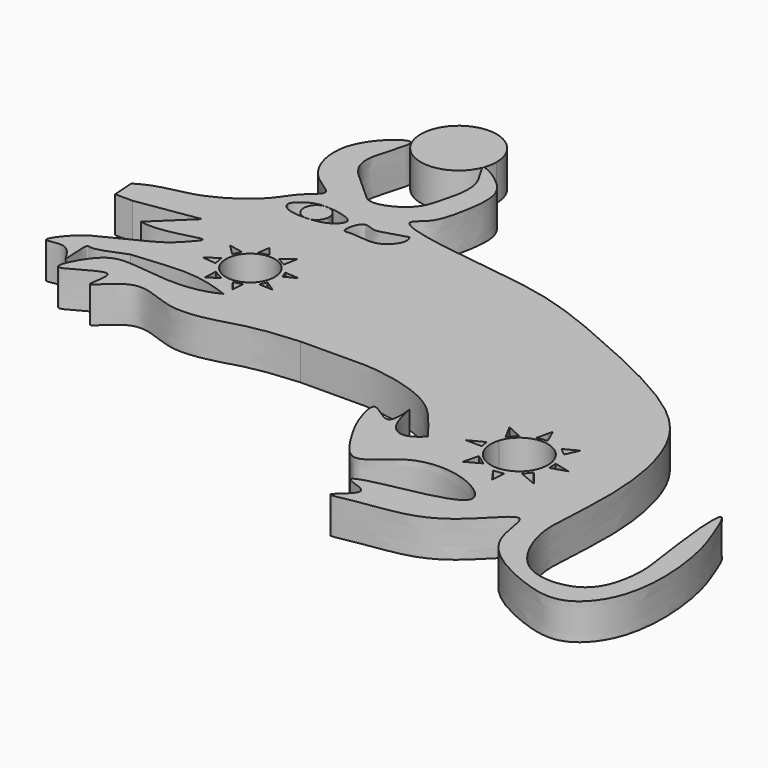
from build123d import *

# Parameters (mm, degrees)
F1_DEPTH = 6.35


with BuildPart() as f1:
    # F0 (on Top) → F1 (new body)
    with BuildSketch(Plane.XY):
        with BuildLine():
            Line((-51.3051622598, 40.6323485076), (-40.4214509814, 42.3343013825))
            Line((-40.4214509814, 42.3343013825), (-46.5386495977, 36.4676751196))
            add(Edge.make_bspline(
                [(-41.5301586996, 27.9514516536), (-43.7644399762, 26.9904386594), (-47.1679695554, 25.6974008069), (-48.0404193502, 26.9466699448), (-47.828587647, 22.82574291), (-47.5278895257, 20.4771889862), (-49.6106092059, 25.4928087476), (-54.8971564778, 22.8735531834), (-51.0068516627, 28.0945899918), (-48.0600885999, 29.6078924967), (-40.1052119231, 33.3394005284), (-38.1358371068, 35.4865499838), (-34.685151176, 39.2845987007), (-42.3593159189, 35.5881020627), (-46.5386495977, 36.4676751196)],
                knots=[0.9023541068, 0.9023541068, 0.9023541068, 0.9023541068, 0.907742959, 0.9125923743, 0.9207853725, 0.9255156021, 0.9337227858, 0.9415669865, 0.9501071173, 0.9590890143, 0.9716437394, 0.9798509262, 0.9862020834, 1, 1, 1, 1], degree=3))
            add(Edge.make_bspline(
                [(-29.9900722132, 33.1400264372), (-34.0198383076, 31.375468556), (-38.2517401569, 29.3615708058), (-41.5301586996, 27.9514516536)],
                knots=[0.8944469051, 0.8944469051, 0.8944469051, 0.8944469051, 0.9023541068, 0.9023541068, 0.9023541068, 0.9023541068], degree=3))
            ThreePointArc((-29.9900722132, 33.1400264372), (-27.7145464501, 39.0940051535), (-22.0091523445, 36.2521117437))
            add(Edge.make_bspline(
                [(-21.3412356287, 36.4475622498), (-21.5580775748, 36.3872225734), (-21.7808652609, 36.3219625695), (-22.0091523444, 36.2521117437)],
                knots=[0.8881591208, 0.8881591208, 0.8881591208, 0.8881591208, 0.8887349681, 0.8887349681, 0.8887349681, 0.8887349681], degree=3))
            Line((-21.3412356287, 36.4475622498), (-21.5400233865, 37.0286330581))
            Line((-21.5400233865, 37.0286330581), (-19.307261154, 36.8855050234))
            add(Edge.make_bspline(
                [(-24.2429566621, 26.7680510879), (-19.3063256589, 29.3490797871), (-14.3387897829, 36.8000169307), (-18.5226528543, 36.9870303006), (-19.307261154, 36.8855050234)],
                knots=[0.8683372636, 0.8683372636, 0.8683372636, 0.8683372636, 0.8834903862, 0.8861495586, 0.8861495586, 0.8861495586, 0.8861495586], degree=3))
            add(Edge.make_bspline(
                [(-7.1130855992, 22.3077908158), (-14.0992043325, 21.8413981828), (-17.6578918044, 20.5122390981), (-27.9317556959, 18.0093599196), (-35.5915896348, 23.5671974151), (-41.853535587, 14.694872303), (-38.2791283301, 24.7989362682), (-49.4655741655, 15.64594504), (-44.996041368, 24.6964345517), (-40.4360164412, 27.0000948649), (-29.9614893405, 23.7782191659), (-24.2429566621, 26.7680510879)],
                knots=[0.7600357456, 0.7600357456, 0.7600357456, 0.7600357456, 0.7751449316, 0.7881314628, 0.800745068, 0.8109455646, 0.8194731054, 0.8310040323, 0.8407808579, 0.8507840727, 0.8683372636, 0.8683372636, 0.8683372636, 0.8683372636], degree=3))
            add(Edge.make_bspline(
                [(36.6513938062, 22.1665031366), (25.3446848612, 23.1486310632), (3.3868181206, 23.0087634058), (-7.1130855992, 22.3077908158)],
                knots=[0.7373271423, 0.7373271423, 0.7373271423, 0.7373271423, 0.7600357456, 0.7600357456, 0.7600357456, 0.7600357456], degree=3))
            Line((36.6513938062, 22.1665031366), (36.8404947221, 22.9985490441))
            Line((36.8404947221, 22.9985490441), (37.2272023111, 22.1146447852))
            add(Edge.make_bspline(
                [(43.3149506831, 20.9869989592), (42.4581897705, 21.4586118414), (40.2700373504, 21.8304625428), (37.2272023111, 22.1146447852)],
                knots=[0.7306147118, 0.7306147118, 0.7306147118, 0.7306147118, 0.7369352057, 0.7369352057, 0.7369352057, 0.7369352057], degree=3))
            Line((43.3149506831, 20.9869989592), (43.3194227517, 20.9893733263))
            Line((43.3194227517, 20.9893733263), (43.3176731158, 20.9854975561))
            add(Edge.make_bspline(
                [(42.7077792689, 19.6344687831), (43.3928146151, 19.9798180502), (43.9528331916, 20.4546398389), (43.5430676641, 20.8609603845), (43.3176731158, 20.9854975561)],
                knots=[0.7254527417, 0.7254527417, 0.7254527417, 0.7254527417, 0.7289397242, 0.7306080061, 0.7306080061, 0.7306080061, 0.7306080061], degree=3))
            Line((42.7077792689, 19.6344687831), (42.2601252794, 18.6428315938))
            Line((42.2601252794, 18.6428315938), (41.6410882083, 19.1666339039))
            add(Edge.make_bspline(
                [(40.5629195083, 18.7687457989), (40.9493693256, 18.9038291277), (41.3108287786, 19.0365662742), (41.6410882083, 19.1666339039)],
                knots=[0.722681181, 0.722681181, 0.722681181, 0.722681181, 0.7239231231, 0.7239231231, 0.7239231231, 0.7239231231], degree=3))
            ThreePointArc((40.5629195083, 18.7687457989), (41.9826037766, 17.0127236479), (42.4899866114, 14.8123418912))
            ThreePointArc((42.4899866114, 14.8123418912), (36.7191210321, 9.8430968264), (32.6616143698, 16.2877012157))
            add(Edge.make_bspline(
                [(24.2925225706, 11.177867651), (25.2786489626, 12.2809637741), (25.9859758486, 13.9796821159), (31.0324810638, 15.7625766968), (32.6616143698, 16.2877012157)],
                knots=[0.701130169, 0.701130169, 0.701130169, 0.701130169, 0.7112861514, 0.7155957737, 0.7155957737, 0.7155957737, 0.7155957737], degree=3))
            add(Edge.make_bspline(
                [(-19.8306408762, 78.5392299294), (-19.4681830159, 78.8542072476), (-14.052009643, 75.6493975615), (-13.0608018564, 71.261285338), (-13.8801468401, 66.2189754635), (-15.0009587895, 61.4008583447), (-19.2283364772, 59.0302462646), (-9.5382100028, 56.3078388494), (9.3444221912, 54.9572718393), (23.6566558066, 49.0942544942), (42.0810289493, 40.7607848748), (51.8920826158, 31.6998617946), (55.4002091748, 16.4829538299), (54.1270442011, 3.0214925536), (54.3000280207, -3.0934207063), (58.9837638875, -12.675226308), (69.9788519865, -11.9014199156), (72.217411324, -5.1737551454), (72.5367364656, 0.2082741773), (70.6239612573, 9.7349605427), (70.0974822964, 20.478680453), (73.1305850924, 12.8140746703), (74.7635899748, 8.3430140955), (76.1863912735, -0.0991630383), (75.3219186096, -10.1324937799), (69.5590091293, -16.6101403474), (61.4090239759, -14.8333269541), (49.6856023234, -8.7620491579), (50.5212507547, 3.0355171184), (43.9292936621, -5.0859771892), (37.6156187166, -9.1681541607), (28.8593361986, -9.890300357), (22.5286818983, -11.5468361423), (29.8147722468, -6.7806682053), (22.1102868722, -5.7114201884), (27.5260276375, -3.5441854087), (44.0455174219, -1.4282130484), (36.946001331, 5.0650103787), (26.2200165544, 6.0766294622), (20.5597810012, -2.4770791815), (15.9981238191, 4.5693886714), (13.4751610374, 9.0111662297), (11.8964872037, 15.6272735635), (18.3266302846, 8.8733808079), (16.7620817514, 19.4488166202), (17.9625657361, 10.9356552545), (21.2681894925, 8.6200225885), (23.5082851271, 10.3006076055), (24.2925225706, 11.177867651)],
                knots=[0.1609755771, 0.1609755771, 0.1609755771, 0.1609755771, 0.1712489865, 0.1807553029, 0.1905404918, 0.2003173152, 0.2074986815, 0.2189418752, 0.2384080978, 0.2559526051, 0.2753237484, 0.2909837027, 0.3079833269, 0.3238509552, 0.3347137649, 0.3480137799, 0.3609716443, 0.3717039637, 0.3817460286, 0.3961976927, 0.4075403835, 0.4168975387, 0.4271996858, 0.4397780643, 0.4536428969, 0.4654112991, 0.4775110011, 0.4931280045, 0.5047246961, 0.5158237941, 0.5284060983, 0.5419012763, 0.5497616364, 0.5586780482, 0.5670500043, 0.5749582402, 0.5913584386, 0.6011184796, 0.6153119041, 0.6271938338, 0.6377176617, 0.6489015976, 0.6571087807, 0.666058114, 0.6752501404, 0.6845896587, 0.6930534136, 0.701130169, 0.701130169, 0.701130169, 0.701130169], degree=3))
            ThreePointArc((-19.8306408762, 78.5392299294), (-19.8514040595, 78.4847419755), (-19.8726420259, 78.4304373192))
            add(Edge.make_bspline(
                [(-54.6811670065, 44.5193760097), (-51.5104317557, 46.5617222984), (-45.6587506237, 46.5226089962), (-37.006843106, 52.1826988629), (-34.9028664648, 56.7072661445), (-30.5837726881, 59.403426729), (-37.4871713574, 61.7908079702), (-40.6390766235, 72.6820217102), (-31.2487696018, 80.3329822257), (-32.8804375491, 74.4464597461), (-35.1583656015, 67.926035361), (-28.1402814143, 63.2079560505), (-25.8142682003, 59.8700914856), (-19.2045932409, 62.8688675297), (-18.1223394986, 67.9704918485), (-16.4824832044, 73.8749221786), (-19.8765539997, 77.9221266737), (-19.8726420259, 78.4304373192)],
                knots=[0, 0, 0, 0, 0.0135520671, 0.0269997263, 0.036979418, 0.0446906139, 0.0544506567, 0.0685807323, 0.0808406192, 0.0887009723, 0.0999473867, 0.1118753668, 0.1201385764, 0.1306354519, 0.1405193258, 0.1516184202, 0.1601742184, 0.1601742184, 0.1601742184, 0.1601742184], degree=3))
            Line((-54.6811670065, 44.5193760097), (-54.4035211205, 40.6323485076))
            Line((-54.4035211205, 40.6323485076), (-51.3051622598, 40.6323485076))
        make_face()
        Polygon((-33.2263410091, 33.4501042962), (-31.102495268, 34.9671393633), (-30.7990889996, 33.2225523889), align=None, mode=Mode.SUBTRACT)
        Polygon((37.6377888024, 8.8067371398), (39.3918305635, 9.0937623754), (39.2004810274, 6.6381008364), align=None, mode=Mode.SUBTRACT)
        Polygon((33.42808038, 10.9753739089), (35.2778024971, 9.6678137779), (32.6945707202, 8.2645788789), align=None, mode=Mode.SUBTRACT)
        Polygon((29.0270261467, 13.5586019605), (31.6421464086, 14.9299455807), (31.865388155, 13.5267106816), align=None, mode=Mode.SUBTRACT)
        Polygon((41.2967503071, 10.5763766915), (42.358674109, 11.8658551946), (44.5204488933, 9.2489719391), align=None, mode=Mode.SUBTRACT)
        Polygon((43.1551150978, 14.2551837489), (43.079264462, 15.8101432025), (45.847851783, 15.1274781674), align=None, mode=Mode.SUBTRACT)
        Polygon((-32.5322896242, 38.6041142046), (-30.0291851163, 38.1110757589), (-30.7118501514, 36.7836728692), align=None, mode=Mode.SUBTRACT)
        Polygon((-26.5077594668, 39.7681519389), (-28.1704533845, 39.2854362726), (-27.8486404568, 41.4844825864), align=None, mode=Mode.SUBTRACT)
        Polygon((-23.1957025826, 38.7657135725), (-24.8265136033, 39.6759323776), (-22.7405913174, 41.306745261), align=None, mode=Mode.SUBTRACT)
        with BuildLine():
            add(Edge.make_bspline(
                [(-29.7085862151, 51.5083821308), (-30.8435993392, 51.4713422911), (-32.9688635459, 51.6536945776), (-34.1280797225, 52.7540945483), (-34.056480974, 53.3193424344)],
                knots=[0.7755982262, 0.7755982262, 0.7755982262, 0.7755982262, 0.898271867, 1, 1, 1, 1], degree=3))
            add(Edge.make_bspline(
                [(-34.056480974, 53.3193424344), (-33.9678045096, 54.0194131062), (-32.0236854991, 55.5713237315), (-30.583744013, 55.8473531372), (-29.7373402864, 55.8715611696)],
                knots=[0, 0, 0, 0, 0.125992302, 0.2438231947, 0.2438231947, 0.2438231947, 0.2438231947], degree=3))
            ThreePointArc((-29.7373402864, 55.8715611696), (-29.3558867656, 55.9014362405), (-28.9749994489, 55.865047227))
            add(Edge.make_bspline(
                [(-28.9749994489, 55.865047227), (-28.1578386624, 55.8296997885), (-26.2794710065, 55.5679093514), (-23.7054649945, 54.5136045418), (-25.6049436606, 52.1402712635), (-27.5666513422, 51.6827797842), (-28.7641105398, 51.569086872)],
                knots=[0.27765671, 0.27765671, 0.27765671, 0.27765671, 0.3824359442, 0.4968478072, 0.6070354314, 0.7410909763, 0.7410909763, 0.7410909763, 0.7410909763], degree=3))
            ThreePointArc((-28.7641105398, 51.569086872), (-29.233059536, 51.48756501), (-29.7085862151, 51.5083821308))
        make_face(mode=Mode.SUBTRACT)
        with BuildLine():
            add(Edge.make_bspline(
                [(-22.2088247538, 54.909735918), (-21.6569007707, 55.3039308839), (-20.1875600639, 54.3732522239), (-18.3712107006, 54.8270045877), (-15.0430986721, 55.8831536711), (-14.7239161253, 55.9909161949), (-14.1242924026, 54.5843781712), (-15.5702228623, 52.3455684269), (-18.0887206373, 51.2089671513), (-21.5689326009, 52.0520055334), (-23.6338879747, 51.3374935701), (-22.9071940869, 54.4109468025), (-22.2088247538, 54.909735918)],
                knots=[0, 0, 0, 0, 0.0969723278, 0.1994822367, 0.3280340651, 0.361375197, 0.4373483182, 0.5480013646, 0.6631276448, 0.7966221843, 0.8772974142, 1, 1, 1, 1], degree=3))
        make_face(mode=Mode.SUBTRACT)
        with BuildLine():
            add(Edge.make_bspline(
                [(-29.9900722132, 33.1400264372), (-34.0198383076, 31.375468556), (-38.2517401569, 29.3615708058), (-41.5301586996, 27.9514516536)],
                knots=[0.8944469051, 0.8944469051, 0.8944469051, 0.8944469051, 0.9023541068, 0.9023541068, 0.9023541068, 0.9023541068], degree=3))
            add(Edge.make_bspline(
                [(-41.5301586996, 27.9514516536), (-37.9919019095, 28.1578397615), (-31.5758020243, 29.2900513337), (-26.1462680998, 27.5211746167), (-24.2429566621, 26.7680510879)],
                knots=[0, 0, 0, 0, 0.5419338711, 1, 1, 1, 1], degree=3))
            add(Edge.make_bspline(
                [(-24.2429566621, 26.7680510879), (-19.3063256589, 29.3490797871), (-14.3387897829, 36.8000169307), (-18.5226528543, 36.9870303006), (-19.307261154, 36.8855050234)],
                knots=[0.8683372636, 0.8683372636, 0.8683372636, 0.8683372636, 0.8834903862, 0.8861495586, 0.8861495586, 0.8861495586, 0.8861495586], degree=3))
            Line((-19.307261154, 36.8855050234), (-19.0524701029, 36.8691720068))
            Line((-19.0524701029, 36.8691720068), (-21.1254302412, 35.8167476952))
            Line((-21.1254302412, 35.8167476952), (-21.3412356287, 36.4475622498))
            add(Edge.make_bspline(
                [(-21.3412356287, 36.4475622498), (-21.5580775748, 36.3872225734), (-21.7808652609, 36.3219625695), (-22.0091523444, 36.2521117437)],
                knots=[0.8881591208, 0.8881591208, 0.8881591208, 0.8881591208, 0.8887349681, 0.8887349681, 0.8887349681, 0.8887349681], degree=3))
            ThreePointArc((-22.0091523445, 36.2521117437), (-21.8883072866, 35.6739408826), (-21.8477710426, 35.0846685469))
            ThreePointArc((-21.8477710426, 35.0846685469), (-25.1514755667, 30.8990174241), (-29.9900722132, 33.1400264372))
        make_face()
        Polygon((-29.2897094041, 28.9919208735), (-29.1940327734, 31.2881246209), (-27.3762065917, 30.2675906569), align=None, mode=Mode.SUBTRACT)
        Polygon((-24.0913592279, 28.5454373807), (-25.4308115691, 30.3313732147), (-23.931901902, 30.6821819395), align=None, mode=Mode.SUBTRACT)
        Polygon((-22.1459660679, 32.0535264909), (-21.6356981546, 33.2335196435), (-19.7221953422, 31.9578498602), align=None, mode=Mode.SUBTRACT)
        with BuildLine():
            add(Edge.make_bspline(
                [(36.6513938062, 22.1665031366), (25.3446848612, 23.1486310632), (3.3868181206, 23.0087634058), (-7.1130855992, 22.3077908158)],
                knots=[0.7373271423, 0.7373271423, 0.7373271423, 0.7373271423, 0.7600357456, 0.7600357456, 0.7600357456, 0.7600357456], degree=3))
            add(Edge.make_bspline(
                [(-7.1130855992, 22.3077908158), (-5.0168499185, 22.3220785179), (-2.6564764721, 22.3221035459), (0.1732082581, 22.2523673446), (5.5379886377, 22.708433948), (18.4827853404, 20.0237589172), (21.9793606491, 13.9566930986), (24.2925225706, 11.177867651)],
                knots=[0, 0, 0, 0, 0.1680254942, 0.29173162, 0.4716710702, 0.7476037536, 1, 1, 1, 1], degree=3))
            add(Edge.make_bspline(
                [(24.2925225706, 11.177867651), (25.2786489626, 12.2809637741), (25.9859758486, 13.9796821159), (31.0324810638, 15.7625766968), (32.6616143698, 16.2877012157)],
                knots=[0.701130169, 0.701130169, 0.701130169, 0.701130169, 0.7112861514, 0.7155957737, 0.7155957737, 0.7155957737, 0.7155957737], degree=3))
            ThreePointArc((32.6616143698, 16.2877012157), (35.9596882525, 19.6064704539), (40.5629195083, 18.7687457989))
            add(Edge.make_bspline(
                [(40.5629195083, 18.7687457989), (40.9493693256, 18.9038291277), (41.3108287786, 19.0365662742), (41.6410882083, 19.1666339039)],
                knots=[0.722681181, 0.722681181, 0.722681181, 0.722681181, 0.7239231231, 0.7239231231, 0.7239231231, 0.7239231231], degree=3))
            Line((41.6410882083, 19.1666339039), (40.9645475447, 19.739093259))
            Line((40.9645475447, 19.739093259), (43.3149506831, 20.9869989592))
            add(Edge.make_bspline(
                [(43.3149506831, 20.9869989592), (42.4581897705, 21.4586118414), (40.2700373504, 21.8304625428), (37.2272023111, 22.1146447852)],
                knots=[0.7306147118, 0.7306147118, 0.7306147118, 0.7306147118, 0.7369352057, 0.7369352057, 0.7369352057, 0.7369352057], degree=3))
            Line((37.2272023111, 22.1146447852), (37.9567034543, 20.4472113401))
            Line((37.9567034543, 20.4472113401), (36.2026616931, 20.1920773834))
            Line((36.2026616931, 20.1920773834), (36.6513938062, 22.1665031366))
        make_face()
        Polygon((31.2913358212, 20.351536572), (33.9702405035, 19.1396512091), (32.7264629304, 17.6726318896), align=None, mode=Mode.SUBTRACT)
        with BuildLine():
            add(Edge.make_bspline(
                [(42.7077792689, 19.6344687831), (43.3928146151, 19.9798180502), (43.9528331916, 20.4546398389), (43.5430676641, 20.8609603845), (43.3176731158, 20.9854975561)],
                knots=[0.7254527417, 0.7254527417, 0.7254527417, 0.7254527417, 0.7289397242, 0.7306080061, 0.7306080061, 0.7306080061, 0.7306080061], degree=3))
            Line((43.3176731158, 20.9854975561), (42.7077792689, 19.6344687831))
        make_face()
    extrude(amount=F1_DEPTH)


with BuildPart() as f1b:
    # F0 (on Top) → F1, piece 2 (new body)
    with BuildSketch(Plane.XY):
        with BuildLine():
            ThreePointArc((-19.403072768, 80.8908417821), (-32.6459937334, 82.143248007), (-19.8726420259, 78.4304373192))
            add(Edge.make_bspline(
                [(-19.8726420259, 78.4304373192), (-19.8722756201, 78.4780470378), (-19.8589137446, 78.5146606947), (-19.8306408762, 78.5392299294)],
                knots=[0.1601742184, 0.1601742184, 0.1601742184, 0.1601742184, 0.1609755771, 0.1609755771, 0.1609755771, 0.1609755771], degree=3))
            ThreePointArc((-19.8306408762, 78.5392299294), (-19.5108339027, 79.6957588569), (-19.403072768, 80.8908417821))
        make_face()
    extrude(amount=F1_DEPTH)


with BuildPart() as f1c:
    # F0 (on Top) → F1, piece 3 (new body)
    with BuildSketch(Plane.XY):
        with BuildLine():
            add(Edge.make_bspline(
                [(-29.7373402864, 55.8715611696), (-29.4943071327, 55.8785121722), (-29.2388630112, 55.8764610162), (-28.9749994489, 55.865047227)],
                knots=[0.2438231947, 0.2438231947, 0.2438231947, 0.2438231947, 0.27765671, 0.27765671, 0.27765671, 0.27765671], degree=3))
            ThreePointArc((-29.7373402864, 55.8715611696), (-31.583965938, 53.6777073348), (-29.7085862151, 51.5083821308))
            add(Edge.make_bspline(
                [(-28.7641105398, 51.569086872), (-28.8264315676, 51.5631697943), (-29.1362873632, 51.5357448895), (-29.4538666354, 51.5166946095), (-29.7085862151, 51.5083821308)],
                knots=[0.7410909763, 0.7410909763, 0.7410909763, 0.7410909763, 0.7480678148, 0.7755982262, 0.7755982262, 0.7755982262, 0.7755982262], degree=3))
            ThreePointArc((-28.7641105398, 51.569086872), (-27.6098450928, 52.3634129184), (-27.1655128285, 53.692266345))
            ThreePointArc((-27.1655128285, 53.692266345), (-27.6771228583, 55.1060572233), (-28.9749994489, 55.865047227))
        make_face()
    extrude(amount=F1_DEPTH)


solid = Compound([f1.part, f1b.part, f1c.part])
